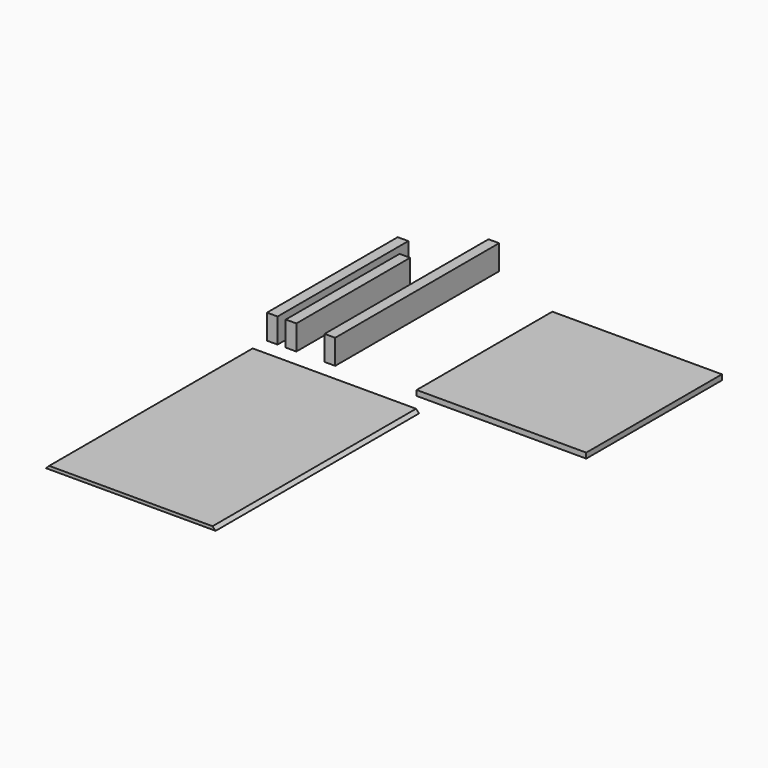
from build123d import *

# Parameters (mm, degrees)
F0_W         = 38.1
F0_H         = 587.375
F1_DEPTH     = 88.9
F2_W         = 38.1
F2_H         = 736.6
F3_DEPTH     = 88.9
F4_W         = 38.1
F4_H         = 511.175
F5_DEPTH     = 88.9
F6_W         = 609.6
F6_H         = 609.6
F7_DEPTH     = 19.05
F8_W         = 609.6
F8_H         = 914.4
F9_DEPTH     = 11.1125
F10_T1_DEPTH = 971.882258147


# Not quite as in the source:
# - a fillet or chamfer that OpenCascade refuses, or shapes differently, is made with other operations: its cross-section is extruded or revolved along the edge and cut away or added
# - a length typed as a fraction of an inch, garbled in the dataset ("3 / 203.2 mm" for 3/8 in), is restored


with BuildPart() as f1:
    # F0 (on Top) → F1 (new body)
    with BuildSketch(Plane.XY):
        with Locations((19.05, 293.6875)):
            Rectangle(F0_W, F0_H)
    extrude(amount=F1_DEPTH)


with BuildPart() as f3:
    # F2 (on Top) → F3 (new body)
    with BuildSketch(Plane.XY):
        with Locations((226.0228706253, 368.3)):
            Rectangle(F2_W, F2_H)
    extrude(amount=F3_DEPTH)


with BuildPart() as f5:
    # F4 (on Top) → F5 (new body)
    with BuildSketch(Plane.XY):
        with Locations((86.4868082545, 255.5875)):
            Rectangle(F4_W, F4_H)
    extrude(amount=F5_DEPTH)


with BuildPart() as f7:
    # F6 (on Top) → F7 (new body)
    with BuildSketch(Plane.XY):
        with Locations((842.7567224306, 304.8)):
            Rectangle(F6_W, F6_H)
    extrude(amount=F7_DEPTH)


with BuildPart() as f9:
    # F8 (on Top) → F9 (new body)
    with BuildSketch(Plane.XY):
        with Locations((304.8, -535.4357879985)):
            Rectangle(F8_W, F8_H)
    extrude(amount=F9_DEPTH)

    # F10: chamfer of 11.176 on 2 edges, made by hand

    # F10_s2 → F10_t1 (cut)
    with BuildSketch(Plane.XZ.offset(49.494658925)):
        Polygon((609.6, -0.0635), (598.424, 11.1125), (609.6, 11.1125), align=None)
        Polygon((0, -0.0635), (11.176, 11.1125), (0, 11.1125), align=None)
    extrude(amount=F10_T1_DEPTH, mode=Mode.SUBTRACT)


solid = Compound([f1.part, f3.part, f5.part, f7.part, f9.part])
